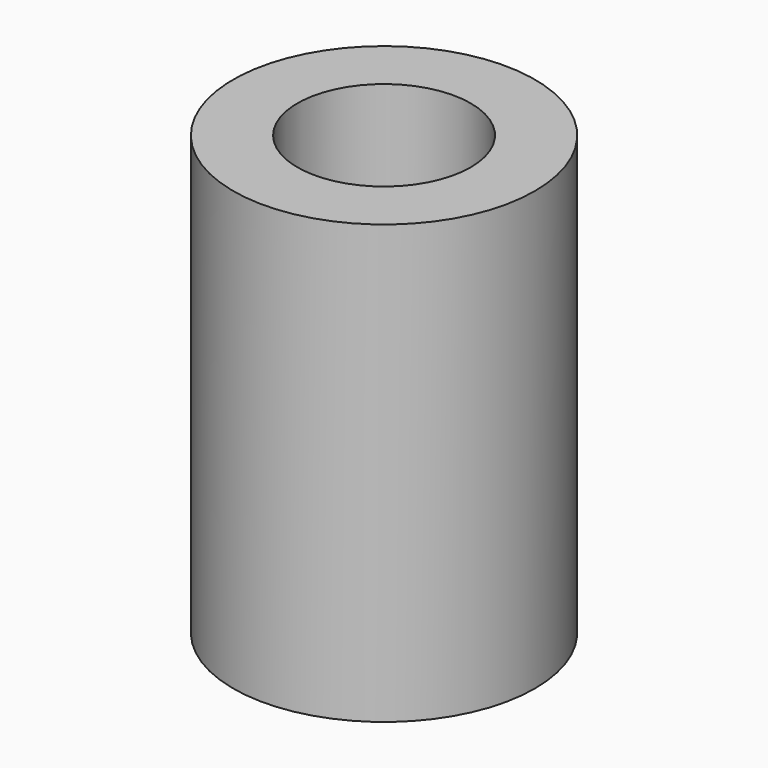
from build123d import *

# Parameters (mm, degrees)
F0_R     = 52.5018
F0_R_2   = 30.1625
F1_DEPTH = 152.4
F3_DEPTH = 52.5028


# Not quite as in the source:
# - a feature names something its author has since deleted; it is built from what else it names


with BuildPart() as f1:
    # F0 (on Top) → F1 (new body)
    with BuildSketch(Plane.XY):
        Circle(F0_R)
        Circle(F0_R_2, mode=Mode.SUBTRACT)
    extrude(amount=-F1_DEPTH)

    # F2 (on Right) → F3 (cut, through all)
    with BuildSketch(Plane.YZ):
        with BuildLine():
            ThreePointArc((0.25, -49.3), (0.1767766953, -49.1232233047), (0, -49.05))
            Line((0, -49.05), (0, -49.55))
            ThreePointArc((0, -49.55), (0.1767766953, -49.4767766953), (0.25, -49.3))
        make_face()
        with BuildLine():
            ThreePointArc((0.25, -103.1), (0.1767766953, -102.9232233047), (0, -102.85))
            Line((0, -102.85), (0, -103.35))
            ThreePointArc((0, -103.35), (0.1767766953, -103.2767766953), (0.25, -103.1))
        make_face()
        with BuildLine():
            Line((0, -103.35), (0, -102.85))
            ThreePointArc((0, -102.85), (-0.25, -103.1), (0, -103.35))
        make_face()
        with BuildLine():
            ThreePointArc((0.25, -100.1), (0.1767766953, -99.9232233047), (0, -99.85))
            Line((0, -99.85), (0, -100.35))
            ThreePointArc((0, -100.35), (0.1767766953, -100.2767766953), (0.25, -100.1))
        make_face()
        with BuildLine():
            Line((0, -100.35), (0, -99.85))
            ThreePointArc((0, -99.85), (-0.25, -100.1), (0, -100.35))
        make_face()
        with BuildLine():
            ThreePointArc((0.25, -52.3), (0.1767766953, -52.1232233047), (0, -52.05))
            Line((0, -52.05), (0, -52.55))
            ThreePointArc((0, -52.55), (0.1767766953, -52.4767766953), (0.25, -52.3))
        make_face()
        with BuildLine():
            Line((0, -52.55), (0, -52.05))
            ThreePointArc((0, -52.05), (-0.25, -52.3), (0, -52.55))
        make_face()
        with BuildLine():
            Line((0, -49.55), (0, -49.05))
            ThreePointArc((0, -49.05), (-0.25, -49.3), (0, -49.55))
        make_face()
    extrude(amount=-F3_DEPTH, mode=Mode.SUBTRACT)


solid = f1.part
